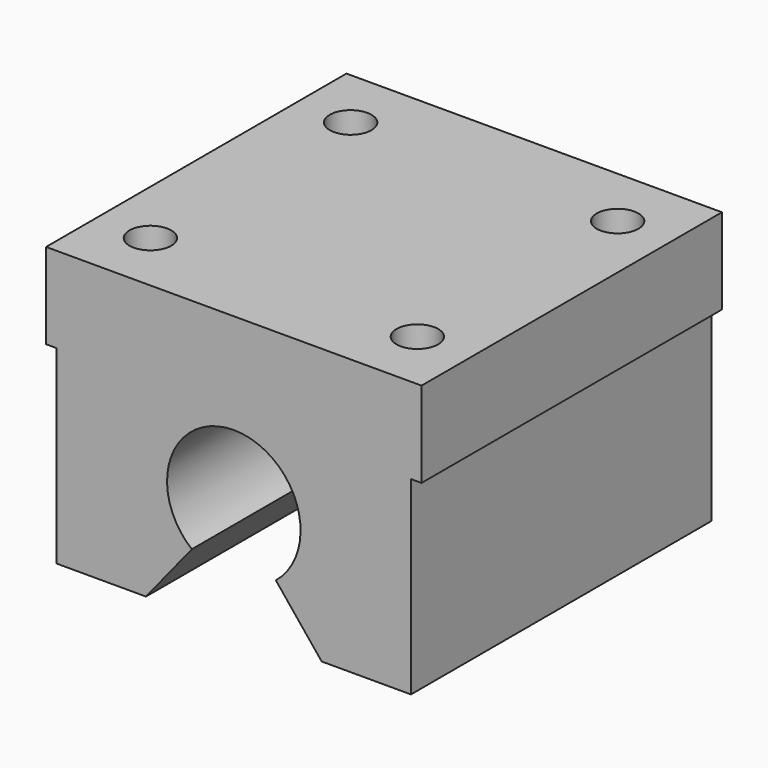
from build123d import *

# Parameters (mm, degrees)
F1_DEPTH = 22.5
F3_START = 12
F2_R     = 2.5
F3_DEPTH = 13


with BuildPart() as f1:
    # F0 (on Front) → F1 (new body, symmetric)
    with BuildSketch(Plane.XZ):
        with BuildLine():
            Line((22.5, 6.23), (22.5, 16.5))
            Line((22.5, 16.5), (-22.5, 16.5))
            Line((-22.5, 16.5), (-22.5, 6.23))
            Line((-22.5, 6.23), (-21.23, 6.23))
            Line((-21.23, 6.23), (-21.23, -16.5))
            Line((-21.23, -16.5), (-10.53, -16.5))
            Line((-10.53, -16.5), (-5.0353739326, -9.7165110278))
            ThreePointArc((-5.0353739326, -9.7165110278), (0, 4.5), (5.0353739326, -9.7165110278))
            Line((5.0353739326, -9.7165110278), (10.53, -16.5))
            Line((10.53, -16.5), (21.23, -16.5))
            Line((21.23, -16.5), (21.23, 6.23))
            Line((21.23, 6.23), (22.5, 6.23))
        make_face()
    extrude(amount=F1_DEPTH, both=True)

    # F2 (on Top) → F3 (cut)
    with BuildSketch(Plane.XY.offset(F3_START)):
        with Locations((-16, 15)):
            Circle(F2_R)
        with Locations((-16, -15)):
            Circle(F2_R)
        with Locations((16, 15)):
            Circle(F2_R)
        with Locations((16, -15)):
            Circle(F2_R)
    extrude(amount=F3_DEPTH, mode=Mode.SUBTRACT)


solid = f1.part
